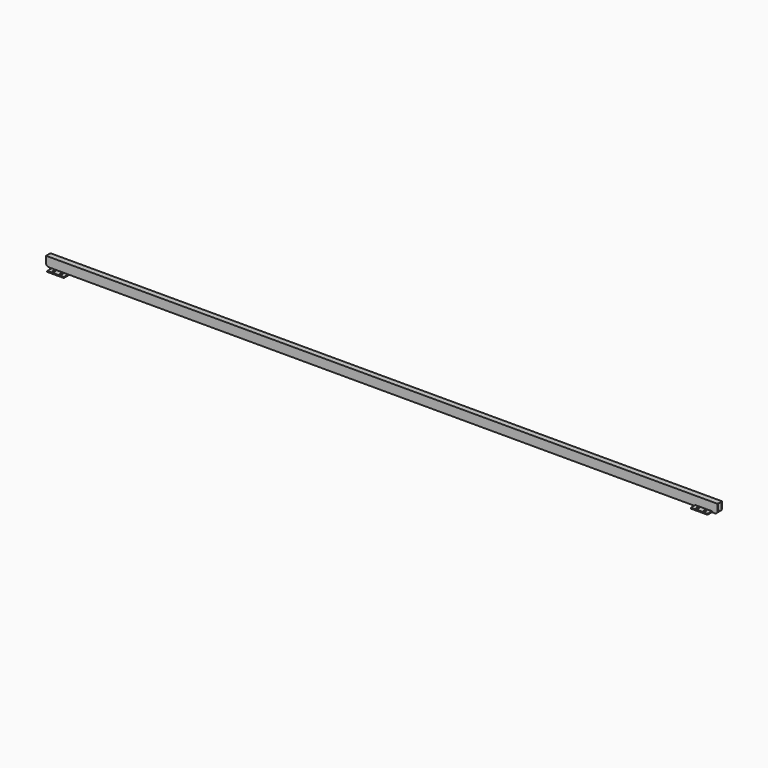
from build123d import *

# Parameters (mm, degrees)
F0_W          = 3575
F0_H          = 50
F1_DEPTH      = 15
F1_DEPTH_BACK = 15
F3_DEPTH      = 5
F5_DEPTH      = 5
F6_R          = 6
F7_DEPTH      = 5
F8_R          = 6
F9_DEPTH      = 5
F12_DEPTH     = 5
F13_W         = 30
F13_H         = 50
F14_DEPTH     = 30
F15_R         = 15
F16_W         = 26
F16_H         = 13
F16_H_2       = 33
F17_DEPTH     = 100
F18_W         = 30
F18_H         = 50
F19_DEPTH     = 30
F20_W         = 26
F20_H         = 46
F21_DEPTH     = 100
F22_T1_DEPTH  = 105
F23_DEPTH     = 5
F24_DEPTH     = 5


# Not quite as in the source:
# - a fillet or chamfer that OpenCascade refuses, or shapes differently, is made with other operations: its cross-section is extruded or revolved along the edge and cut away or added


with BuildPart() as f1:
    # F0 (on Front) → F1 (new body, two sides)
    with BuildSketch(Plane.XZ) as f1_sk:
        Rectangle(F0_W, F0_H)
    extrude(amount=F1_DEPTH)
    extrude(f1_sk.sketch, amount=-F1_DEPTH_BACK)

    # F2 (on face) → F3 (join)
    with BuildSketch(Plane(origin=(0, 0, -25), x_dir=(1, 0, 0), z_dir=(0, 0, -1))):
        Polygon((-1787.5, 45), (-1787.5, 15), (-1787.5, -15), (-1697.5, -15), (-1697.5, 45), align=None)
    extrude(amount=F3_DEPTH)

    # F4 (on face) → F5 (join)
    with BuildSketch(Plane(origin=(0, 0, -25), x_dir=(1, 0, 0), z_dir=(0, 0, -1))):
        Polygon((1787.5, -15), (1787.5, 15), (1787.5, 45), (1697.5, 45), (1697.5, -15), align=None)
    extrude(amount=F5_DEPTH)

    # F6 (on face) → F7 (cut, through all)
    with BuildSketch(Plane(origin=(0, 0, -30), x_dir=(1, 0, 0), z_dir=(0, 0, -1))):
        with Locations((-935, 30)):
            Circle(F6_R)
        with Locations((-975, 30)):
            Circle(F6_R)
    extrude(amount=-F7_DEPTH, mode=Mode.SUBTRACT)

    # F8 (on face) → F9 (cut, through all)
    with BuildSketch(Plane(origin=(0, 0, -30), x_dir=(1, 0, 0), z_dir=(0, 0, -1))):
        with Locations((1762.5, 30)):
            Circle(F8_R)
        with Locations((1722.5, 30)):
            Circle(F8_R)
    extrude(amount=-F9_DEPTH, mode=Mode.SUBTRACT)

    # F11 (on face) → F12 (cut, through all)
    with BuildSketch(Plane(origin=(0, 0, -30), x_dir=(1, 0, 0), z_dir=(0, 0, -1))):
        with BuildLine():
            ThreePointArc((-1762.5, 36), (-1766.7426406871, 34.2426406871), (-1768.5, 30))
            Line((-1768.5, 30), (-1762.5, 30))
            Line((-1762.5, 30), (-1762.5, 36))
        make_face()
        with BuildLine():
            ThreePointArc((-1716.5, 30), (-1722.5, 36), (-1728.5, 30))
            ThreePointArc((-1728.5, 30), (-1722.5, 24), (-1716.5, 30))
        make_face()
        with BuildLine():
            Line((-1762.5, 30), (-1768.5, 30))
            ThreePointArc((-1768.5, 30), (-1762.5, 24), (-1756.5, 30))
            Line((-1756.5, 30), (-1762.5, 30))
        make_face()
        with BuildLine():
            Line((-1762.5, 36), (-1762.5, 30))
            Line((-1762.5, 30), (-1756.5, 30))
            ThreePointArc((-1756.5, 30), (-1758.2573593129, 34.2426406871), (-1762.5, 36))
        make_face()
    extrude(amount=-F12_DEPTH, mode=Mode.SUBTRACT)

    # F13 (on face) → F14 (join)
    with BuildSketch(Plane.YZ.offset(1787.5)):
        Rectangle(F13_W, F13_H)
    extrude(amount=F14_DEPTH)

    # F15
    f15_edges = [f1.edges().sort_by_distance(p)[0] for p in [
        (1817.5, 0, -25),
    ]]
    fillet(f15_edges, radius=F15_R)

    # F16 (on face) → F17 (cut)
    with BuildSketch(Plane.YZ.offset(1817.5)):
        with Locations((0, -16.5)):
            Rectangle(F16_W, F16_H)
        with Locations((0, 6.5)):
            Rectangle(F16_W, F16_H_2)
    extrude(amount=-F17_DEPTH, mode=Mode.SUBTRACT)

    # F18 (on face) → F19 (join)
    with BuildSketch(Plane(origin=(-1787.5, 0, 0), x_dir=(0, -1, 0), z_dir=(-1, 0, 0))):
        Rectangle(F18_W, F18_H)
    extrude(amount=F19_DEPTH)

    # F20 (on face) → F21 (cut)
    with BuildSketch(Plane(origin=(-1817.5, 0, 0), x_dir=(0, -1, 0), z_dir=(-1, 0, 0))):
        Rectangle(F20_W, F20_H)
    extrude(amount=-F21_DEPTH, mode=Mode.SUBTRACT)

    # F22: fillet of radius 15 on 1 edges, made by hand

    # F22_s2 → F22_t1 (cut)
    with BuildSketch(Plane.XZ.offset(-52.5)):
        with BuildLine():
            ThreePointArc((-1817.5, -10), (-1813.1066017178, -20.6066017178), (-1802.5, -25))
            Line((-1802.5, -25), (-1817.5, -25))
            Line((-1817.5, -25), (-1817.5, -10))
        make_face()
    extrude(amount=F22_T1_DEPTH, mode=Mode.SUBTRACT)

    # F23 (add): a face of the model
    f23_faces = [f1.faces().sort_by_distance(p)[0] for p in [
        (1742.5, -30, -25),
    ]]
    extrude(f23_faces, amount=F23_DEPTH)

    # F24 (cut): a face of the model
    f24_faces = [f1.faces().sort_by_distance(p)[0] for p in [
        (1742.5, -14.3442118808, -30),
    ]]
    extrude(f24_faces, amount=-F24_DEPTH, mode=Mode.SUBTRACT)


solid = f1.part
